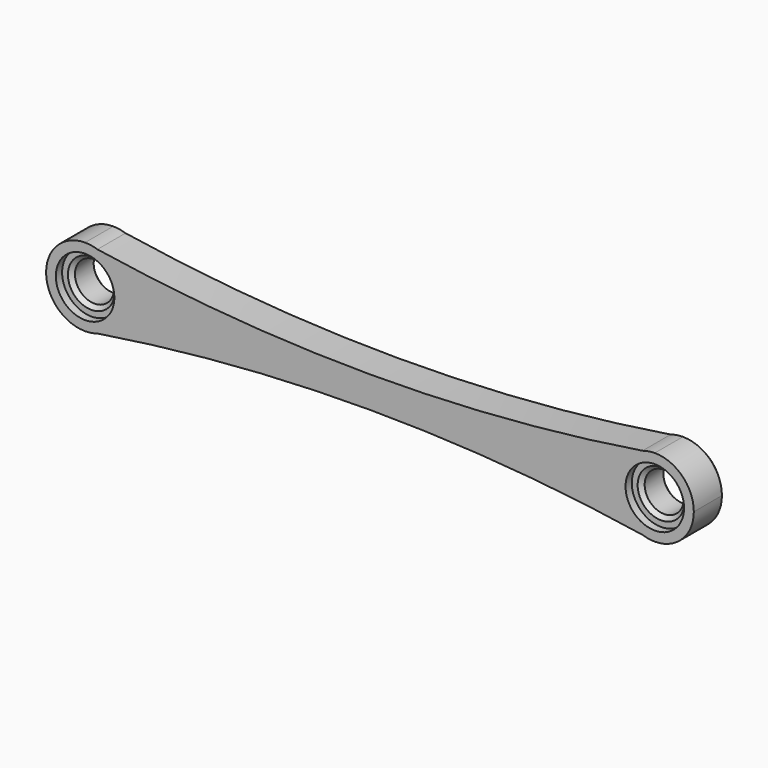
from build123d import *

# Parameters (mm, degrees)
F0_R       = 5
F1_DEPTH   = 10
F2_R       = 7.5
F3_DEPTH   = 2
F4_C1_SIZE = 1
F4_C2_SIZE = 1
F4_C3_SIZE = 1
F4_C4_SIZE = 1
F4_C5_SIZE = 1
F4_C6_SIZE = 1
F4_C7_SIZE = 0.9999
F4_C8_SIZE = 1


# Not quite as in the source:
# - a fillet or chamfer is up to 0.001 mm smaller than in the source, because OpenCascade refuses the exact size


with BuildPart() as f1:
    # F0 (on Front) → F1 (new body)
    with BuildSketch(Plane.XZ):
        with BuildLine():
            ThreePointArc((3.1540486056, 9.4895720343), (1.5765683293, 9.7419684548), (0, 10))
            ThreePointArc((0, 10), (-10, 0), (0, -10))
            ThreePointArc((0, -10), (1.5765683293, -9.7419684548), (3.1540486056, -9.4895720343))
            ThreePointArc((3.1540486056, -9.4895720343), (8.1098855126, -5.8506202211), (10, 0))
            ThreePointArc((10, 0), (8.1098855126, 5.8506202211), (3.1540486056, 9.4895720343))
        make_face()
        Circle(F0_R, mode=Mode.SUBTRACT)
        with BuildLine():
            ThreePointArc((3.1540486056, 9.4895720343), (1.5975418081, 9.8715682731), (0, 10))
            ThreePointArc((0, 10), (1.5765683293, 9.7419684548), (3.1540486056, 9.4895720343))
        make_face()
        with BuildLine():
            ThreePointArc((3.1540486056, -9.4895720343), (1.5765683293, -9.7419684548), (0, -10))
            ThreePointArc((0, -10), (1.5975418081, -9.8715682731), (3.1540486056, -9.4895720343))
        make_face()
        with BuildLine():
            ThreePointArc((142.8459513944, 9.4895720343), (73, 4), (3.1540486056, 9.4895720343))
            ThreePointArc((3.1540486056, 9.4895720343), (8.1098855126, 5.8506202211), (10, 0))
            ThreePointArc((10, 0), (8.1098855126, -5.8506202211), (3.1540486056, -9.4895720343))
            ThreePointArc((3.1540486056, -9.4895720343), (73, -4), (142.8459513944, -9.4895720343))
            ThreePointArc((142.8459513944, -9.4895720343), (136, 0), (142.8459513944, 9.4895720343))
        make_face()
        with BuildLine():
            ThreePointArc((146, 10), (144.4234316707, 9.7419684548), (142.8459513944, 9.4895720343))
            ThreePointArc((142.8459513944, 9.4895720343), (136, 0), (142.8459513944, -9.4895720343))
            ThreePointArc((142.8459513944, -9.4895720343), (144.4234316707, -9.7419684548), (146, -10))
            ThreePointArc((146, -10), (153.0710678119, -7.0710678119), (156, 0))
            ThreePointArc((156, 0), (153.0710678119, 7.0710678119), (146, 10))
        make_face()
        with Locations((146, 0)):
            Circle(F0_R, mode=Mode.SUBTRACT)
        with BuildLine():
            ThreePointArc((146, 10), (144.4024581919, 9.8715682731), (142.8459513944, 9.4895720343))
            ThreePointArc((142.8459513944, 9.4895720343), (144.4234316707, 9.7419684548), (146, 10))
        make_face()
        with BuildLine():
            ThreePointArc((146, -10), (144.4234316707, -9.7419684548), (142.8459513944, -9.4895720343))
            ThreePointArc((142.8459513944, -9.4895720343), (144.4024581919, -9.8715682731), (146, -10))
        make_face()
    extrude(amount=F1_DEPTH)

    # F2 (on face) → F3 (cut)
    with BuildSketch(Plane.XZ.offset(10)):
        Circle(F2_R)
        with Locations((146, 0)):
            Circle(F2_R)
    extrude(amount=-F3_DEPTH, mode=Mode.SUBTRACT)

    # F4: chamfer of 1 on 8 edges, made by hand

    # F4_c1
    f4_c1_edges = [f1.edges().sort_by_distance(p)[0] for p in [
        (73, 0, -4),
    ]]
    chamfer(f4_c1_edges, length=F4_C1_SIZE)

    # F4_c2
    f4_c2_edges = [f1.edges().sort_by_distance(p)[0] for p in [
        (73, 0, 3.9999999999),
    ]]
    chamfer(f4_c2_edges, length=F4_C2_SIZE)

    # F4_c3
    f4_c3_edges = [f1.edges().sort_by_distance(p)[0] for p in [
        (-5, 0, 0),
    ]]
    chamfer(f4_c3_edges, length=F4_C3_SIZE)

    # F4_c4
    f4_c4_edges = [f1.edges().sort_by_distance(p)[0] for p in [
        (141, 0, 0),
    ]]
    chamfer(f4_c4_edges, length=F4_C4_SIZE)

    # F4_c5
    f4_c5_edges = [f1.edges().sort_by_distance(p)[0] for p in [
        (-5, -8, 0),
    ]]
    chamfer(f4_c5_edges, length=F4_C5_SIZE)

    # F4_c6
    f4_c6_edges = [f1.edges().sort_by_distance(p)[0] for p in [
        (141, -8, 0),
    ]]
    chamfer(f4_c6_edges, length=F4_C6_SIZE)

    # F4_c7 (size 1 in the source; OpenCascade refuses exactly that, so slightly less here)
    f4_c7_edges = [f1.edges().sort_by_distance(p)[0] for p in [
        (-10, 0, 0),
    ]]
    chamfer(f4_c7_edges, length=F4_C7_SIZE)

    # F4_c8
    f4_c8_edges = [f1.edges().sort_by_distance(p)[0] for p in [
        (156, 0, 0),
    ]]
    chamfer(f4_c8_edges, length=F4_C8_SIZE)


solid = f1.part
